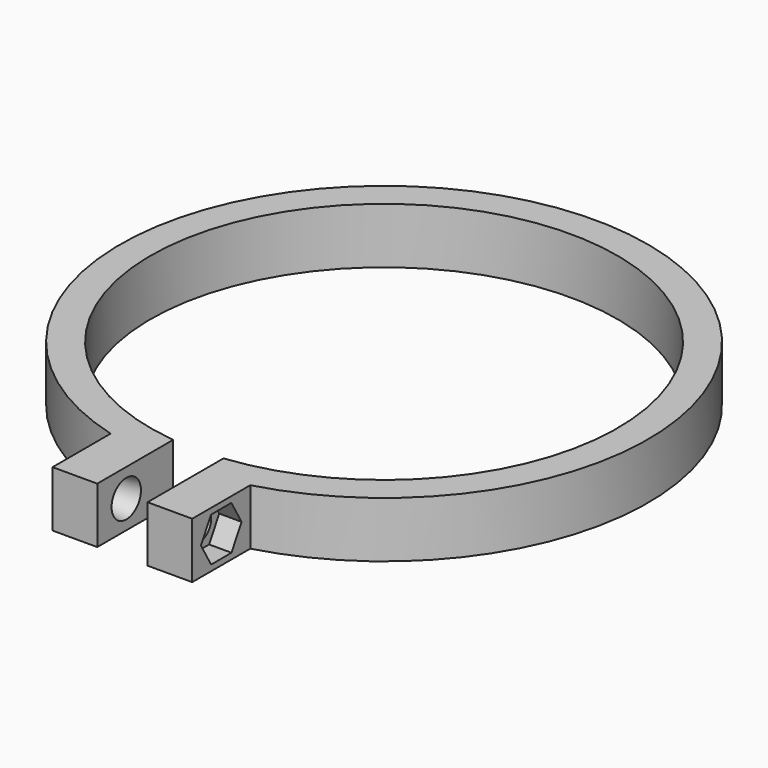
from build123d import *

# Parameters (mm, degrees)
F0_R      = 47.25
F0_R_2    = 41.8
F1_DEPTH  = 10
F2_W      = 4.5
F2_H      = 12.6647017896
F3_DEPTH  = 25
F4_W      = 8
F4_H      = 17
F5_DEPTH  = 10
F7_DEPTH  = 4
F8_R      = 2.55
F9_DEPTH  = 25
F10_SIZE2 = 6
F10_SIZE  = 0.7367073654


# Not quite as in the source:
# - a fillet or chamfer that OpenCascade refuses, or shapes differently, is made with other operations: its cross-section is extruded or revolved along the edge and cut away or added


with BuildPart() as f1:
    # F0 (on Top) → F1 (new body)
    with BuildSketch(Plane.XY):
        Circle(F0_R)
        Circle(F0_R_2, mode=Mode.SUBTRACT)
    extrude(amount=F1_DEPTH)

    # F2 (on Top) → F3 (cut)
    with BuildSketch(Plane.XY):
        with Locations((-2.25, -45.0298693031)):
            Rectangle(F2_W, F2_H)
        with Locations((2.25, -45.0298693031)):
            Rectangle(F2_W, F2_H)
    extrude(amount=F3_DEPTH, mode=Mode.SUBTRACT)

    # F4 (on Top) → F5 (join)
    with BuildSketch(Plane.XY):
        with Locations((8.5, -50.0570691941)):
            Rectangle(F4_W, F4_H)
        with Locations((-8.5, -50.0570691941)):
            Rectangle(F4_W, F4_H)
    extrude(amount=F5_DEPTH)

    # F6 (on face) → F7 (cut)
    with BuildSketch(Plane.YZ.offset(12.5)):
        Polygon((-49.7724240202, 1.0679314721), (-47.5118511184, 5.0166414077), (-49.8012477839, 8.9487099356), (-54.3512173512, 8.9320685279), (-56.6117902531, 4.9833585923), (-54.3223935876, 1.0512900644), align=None)
    extrude(amount=-F7_DEPTH, mode=Mode.SUBTRACT)

    # F8 (on face) → F9 (cut)
    with BuildSketch(Plane.YZ.offset(8.5)):
        with Locations((-52.0618206857, 5)):
            Circle(F8_R)
    extrude(amount=-F9_DEPTH, mode=Mode.SUBTRACT)

    # F10
    f10_edges = [f1.edges().sort_by_distance(p)[0] for p in [
        (-4.5, -54.611821, 5),
    ]]
    f10_side = f1.faces().sort_by_distance((-4.5, -50.057069, 0.197231))[0]
    chamfer(f10_edges, length=F10_SIZE, length2=F10_SIZE2, reference=f10_side)

    # F11: chamfer of 6 x 0.6306254116 on 1 edges, made by hand

    # F11_s1 → F11_t2 (revolve, cut)
    with BuildSketch(Plane.XY.offset(5)):
        Polygon((4.5, -48.8811952741), (10.5, -49.5118206857), (4.5, -49.5118206857), align=None)
    revolve(axis=Axis((4.5, -52.0618206857, 5), (1, 0, 0)), mode=Mode.SUBTRACT)


solid = f1.part
